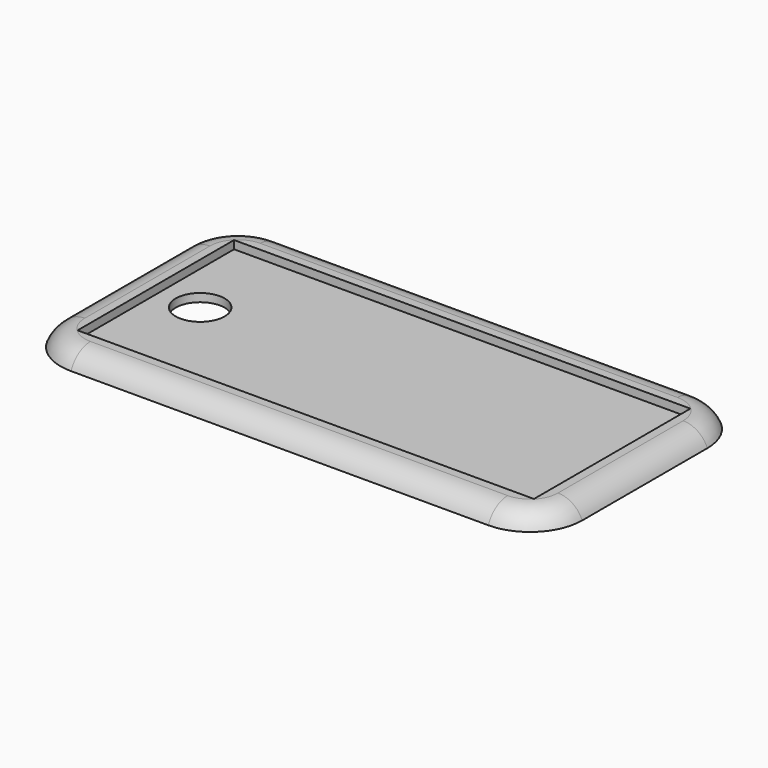
from build123d import *

# Parameters (mm, degrees)
F0_W         = 44.45
F0_H         = 19.05
F0_R         = 2.38125
F1_DEPTH     = 0.79375
F0_W_2       = 50.8
F0_H_2       = 25.4
F2_DEPTH     = 1.5875
F3_R         = 5.08
F4_T1_DEPTH  = 40.64
F4_T3_DEPTH  = 15.24
F4_T6_ANGLE  = 90
F4_T8_ANGLE  = 90
F4_T10_ANGLE = 90
F4_T12_ANGLE = 90
F5_TEXT_SIZE = 18.6560229243
F6_DEPTH     = 0.79375


# Not quite as in the source:
# - a fillet or chamfer that OpenCascade refuses, or shapes differently, is made with other operations: its cross-section is extruded or revolved along the edge and cut away or added
# - a length typed as a fraction of an inch, garbled in the dataset ("3 / 203.2 mm" for 3/8 in), is restored
# - Text() gives the source's letters only with a copy of the font that has no kerning and outlines rounded to 1/6400 em; it was checked with that copy


with BuildPart() as f1:
    # F0 (on Top) → F1 (new body)
    with BuildSketch(Plane.XY):
        with Locations((25.4, 12.7)):
            Rectangle(F0_W, F0_H)
        with Locations((7.14375, 13.1403291598)):
            Circle(F0_R, mode=Mode.SUBTRACT)
    extrude(amount=F1_DEPTH)

    # F0 (on Top) → F2 (join)
    with BuildSketch(Plane.XY):
        with Locations((25.4, 12.7)):
            Rectangle(F0_W_2, F0_H_2)
        with Locations((25.4, 12.7)):
            Rectangle(F0_W, F0_H, mode=Mode.SUBTRACT)
    extrude(amount=F2_DEPTH)

    # F3
    f3_edges = [f1.edges().sort_by_distance(p)[0] for p in [
        (50.8, 0, 0.79375),
        (50.8, 25.4, 0.79375),
        (0, 0, 0.79375),
        (0, 25.4, 0.79375),
    ]]
    fillet(f3_edges, radius=F3_R)

    # F4: fillet of radius 2.54 on 1 edges, made by hand

    # F4_s2 → F4_t1 (cut)
    with BuildSketch(Plane.YZ.offset(5.08)):
        with BuildLine():
            ThreePointArc((0, 0), (0.9347398539, 1.1535567419), (2.3546430197, 1.5875))
            Line((2.3546430197, 1.5875), (0, 1.5875))
            Line((0, 1.5875), (0, 0))
        make_face()
        with BuildLine():
            ThreePointArc((25.4, 0), (24.4652601461, 1.1535567419), (23.0453569803, 1.5875))
            Line((23.0453569803, 1.5875), (25.4, 1.5875))
            Line((25.4, 1.5875), (25.4, 0))
        make_face()
    extrude(amount=F4_T1_DEPTH, mode=Mode.SUBTRACT)

    # F4_s4 → F4_t3 (cut)
    with BuildSketch(Plane.XZ.offset(-20.32)):
        with BuildLine():
            ThreePointArc((50.8, 0), (49.8652601461, 1.1535567419), (48.4453569803, 1.5875))
            Line((48.4453569803, 1.5875), (50.8, 1.5875))
            Line((50.8, 1.5875), (50.8, 0))
        make_face()
        with BuildLine():
            ThreePointArc((0, 0), (0.9347398539, 1.1535567419), (2.3546430197, 1.5875))
            Line((2.3546430197, 1.5875), (0, 1.5875))
            Line((0, 1.5875), (0, 0))
        make_face()
    extrude(amount=F4_T3_DEPTH, mode=Mode.SUBTRACT)

    # F4_s5 → F4_t6 (revolve, cut)
    with BuildSketch(Plane.XZ.offset(-5.08)):
        with BuildLine():
            ThreePointArc((0, 0), (0.9347398539, 1.1535567419), (2.3546430197, 1.5875))
            Line((2.3546430197, 1.5875), (0, 1.5875))
            Line((0, 1.5875), (0, 0))
        make_face()
    revolve(axis=Axis((5.08, 5.08, 1.5875), (0, 0, 1)), revolution_arc=F4_T6_ANGLE, mode=Mode.SUBTRACT)

    # F4_s7 → F4_t8 (revolve, cut)
    with BuildSketch(Plane.YZ.offset(45.72)):
        with BuildLine():
            ThreePointArc((0, 0), (0.9347398539, 1.1535567419), (2.3546430197, 1.5875))
            Line((2.3546430197, 1.5875), (0, 1.5875))
            Line((0, 1.5875), (0, 0))
        make_face()
    revolve(axis=Axis((45.72, 5.08, 1.5875), (0, 0, 1)), revolution_arc=F4_T8_ANGLE, mode=Mode.SUBTRACT)

    # F4_s9 → F4_t10 (revolve, cut)
    with BuildSketch(Plane.YZ.offset(45.72)):
        with BuildLine():
            ThreePointArc((25.4, 0), (24.4652601461, 1.1535567419), (23.0453569803, 1.5875))
            Line((23.0453569803, 1.5875), (25.4, 1.5875))
            Line((25.4, 1.5875), (25.4, 0))
        make_face()
    revolve(axis=Axis((45.72, 20.32, 1.5875), (0, 0, -1)), revolution_arc=F4_T10_ANGLE, mode=Mode.SUBTRACT)

    # F4_s11 → F4_t12 (revolve, cut)
    with BuildSketch(Plane.YZ.offset(5.08)):
        with BuildLine():
            ThreePointArc((25.4, 0), (24.4652601461, 1.1535567419), (23.0453569803, 1.5875))
            Line((23.0453569803, 1.5875), (25.4, 1.5875))
            Line((25.4, 1.5875), (25.4, 0))
        make_face()
    revolve(axis=Axis((5.08, 20.32, 1.5875), (0, 0, 1)), revolution_arc=F4_T12_ANGLE, mode=Mode.SUBTRACT)

    # F5 (on Top) → F6 (join)
    with BuildSketch(Plane.XY):
        with Locations((11.3882860169, 5.9374817647)):
            Text('Joe', F5_TEXT_SIZE, font='Open Sans', font_style=FontStyle.BOLDITALIC, text_align=(TextAlign.LEFT, TextAlign.BOTTOM))
    extrude(amount=F6_DEPTH)


solid = f1.part
